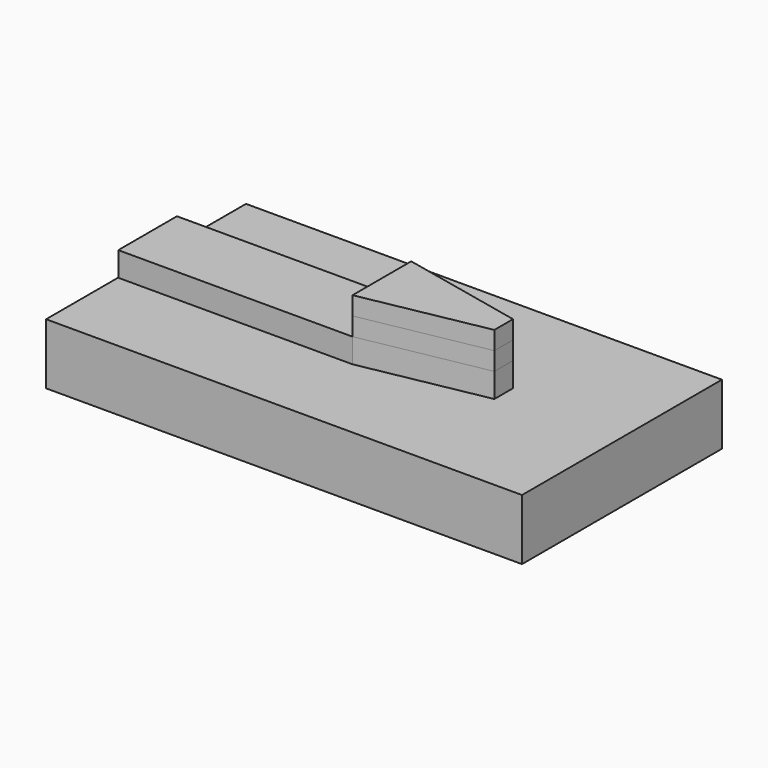
from build123d import *

# Parameters (mm, degrees)
F0_W     = 198.6827738583
F0_H     = 104.3191924691
F1_DEPTH = 25.4
F3_DEPTH = 10.16
F5_DEPTH = 7.62
F7_DEPTH = 7.62


# Not quite as in the source:
# - a feature names something its author has since deleted; it is built from what else it names


with BuildPart() as f1:
    # F0 (on Top) → F1 (new body)
    with BuildSketch(Plane.XY):
        with Locations((-49.9562527984, 0)):
            Rectangle(F0_W, F0_H)
    extrude(amount=-F1_DEPTH)


with BuildPart() as f3:
    # F2 (on face) → F3 (new body)
    with BuildSketch(Plane.XY):
        Polygon((0, 4.8675285652), (-51.4132715762, 16.0222817212), (-149.2118090391, 16.0222817212), (-149.2118090391, -14.602586627), (-51.4132715762, -14.602586627), (0, -4.8675285652), align=None)
    extrude(amount=F3_DEPTH)


with BuildPart() as f5:
    # F4 (on face) → F5 (new body)
    with BuildSketch(Plane.XY.offset(10.16)):
        Polygon((0, 4.8675285652), (-51.4132715762, 16.0222817212), (-51.4132715762, -14.602586627), (0, -4.8675285652), align=None)
    extrude(amount=F5_DEPTH)


with BuildPart() as f7:
    # F6 (on face) → F7 (new body)
    with BuildSketch(Plane.XY.offset(17.78)):
        Polygon((0, 4.8675285652), (-51.4132715762, 16.0222817212), (-51.4132715762, -14.602586627), (0, -4.8675285652), align=None)
    extrude(amount=F7_DEPTH)


solid = Compound([f1.part, f3.part, f5.part, f7.part])
